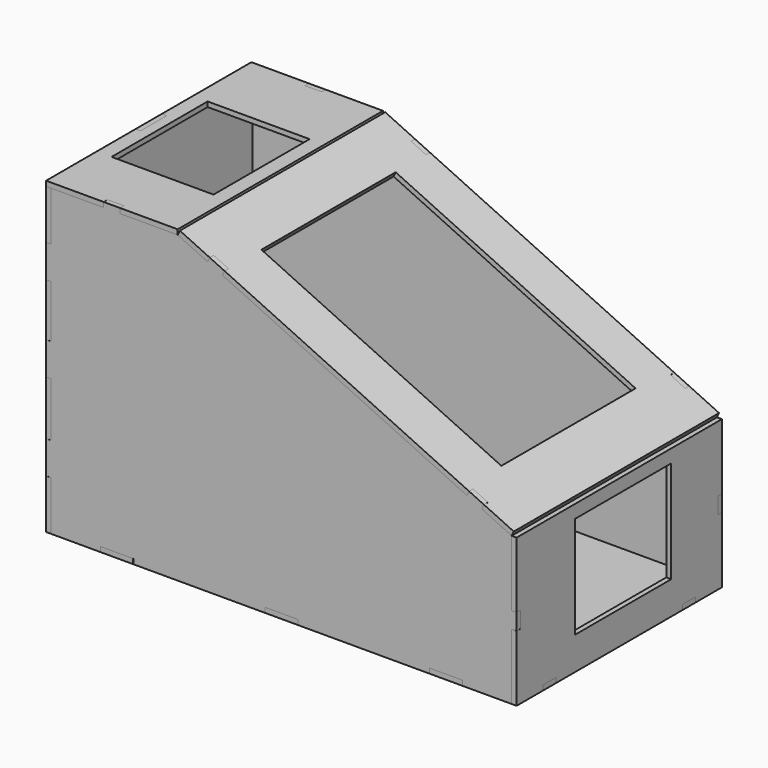
from build123d import *

# Parameters (mm, degrees)
F0_W      = 280
F0_H      = 150
F1_DEPTH  = 3
F2_W      = 73
F2_H      = 62
F2_W_2    = 17
F2_H_2    = 3
F2_W_3    = 96
F3_DEPTH  = 3
F4_W      = 27
F4_H      = 3
F4_W_2    = 66
F4_W_3    = 17
F5_DEPTH  = 3
F6_W      = 3
F6_H      = 68
F6_W_2    = 62
F6_H_2    = 73
F7_DEPTH  = 3
F8_W      = 280
F8_H      = 3
F9_DEPTH  = 3
F10_W     = 280
F10_H     = 3
F11_DEPTH = 3
F12_W     = 20
F12_H     = 3
F12_W_2   = 164.0647657623
F12_W_3   = 161
F12_H_2   = 102
F13_DEPTH = 3
F14_W     = 3
F14_H     = 19.9761795811
F15_DEPTH = 3
F16_W     = 3
F16_H     = 19.9768692255
F16_H_2   = 19.9654474854
F16_H_3   = 19.9758000672
F17_DEPTH = 3
F18_W     = 19.950363785
F18_H     = 3
F18_W_2   = 19.9684463441
F19_DEPTH = 3
F20_W     = 3
F20_H     = 19.9769586325
F20_H_2   = 19.9680477381
F20_H_3   = 19.977606833
F21_DEPTH = 3
F23_W     = 9.9835321307
F23_H     = 3
F24_DEPTH = 3
F25_W     = 9.978748858
F25_H     = 3
F26_DEPTH = 3
F27_W     = 20
F27_H     = 3
F28_DEPTH = 3
F29_W     = 20
F29_H     = 3
F30_DEPTH = 3
F31_W     = 19.9709534645
F31_H     = 3
F31_W_2   = 19.9618935585
F31_W_3   = 19.9760207906
F32_DEPTH = 3
F33_W     = 9.9784359336
F33_H     = 3
F33_W_2   = 9.994674474
F34_DEPTH = 3
F35_W     = 3
F35_H     = 9.9887661636
F36_DEPTH = 3
F37_W     = 3
F37_H     = 9.9958628416
F38_DEPTH = 3
F39_W     = 19.973538816
F39_H     = 3
F39_W_2   = 19.9738545343
F39_W_3   = 19.9763923883
F40_DEPTH = 3
F41_W     = 9.9856257439
F41_H     = 3
F41_W_2   = 9.9614001811
F42_DEPTH = 3
F43_W     = 9.9793635309
F43_H     = 3
F43_W_2   = 9.9839419127
F44_DEPTH = 3


with BuildPart() as f1:
    # F0 (on Top) → F1 (new body)
    with BuildSketch(Plane.XY):
        with Locations((0.3347266465, 5.760698552)):
            Rectangle(F0_W, F0_H)
    extrude(amount=F1_DEPTH)

    # F18 (on face) → F19 (join)
    with BuildSketch(Plane(origin=(-139.6652733535, 0, 0), x_dir=(0, -1, 0), z_dir=(-1, 0, 0))):
        with Locations((-53.7553559989, 1.5)):
            Rectangle(F18_W, F18_H)
        with Locations((32.2464499623, 1.5)):
            Rectangle(F18_W_2, F18_H)
    extrude(amount=F19_DEPTH)

    # F31 (on face) → F32 (join)
    with BuildSketch(Plane.XZ.offset(69.239301448)):
        with Locations((-99.6759831905, 1.5)):
            Rectangle(F31_W, F31_H)
        with Locations((100.318454206, 1.5)):
            Rectangle(F31_W_2, F31_H)
        with Locations((0.3386368044, 1.5)):
            Rectangle(F31_W_3, F31_H)
    extrude(amount=F32_DEPTH)

    # F33 (on face) → F34 (join)
    with BuildSketch(Plane.YZ.offset(140.3347266465)):
        with Locations((-47.2331680357, 1.5)):
            Rectangle(F33_W, F33_H)
        with Locations((58.7589647621, 1.5)):
            Rectangle(F33_W_2, F33_H)
    extrude(amount=F34_DEPTH)

    # F39 (on face) → F40 (join)
    with BuildSketch(Plane(origin=(0, 80.760698552, 0), x_dir=(-1, 0, 0), z_dir=(0, 1, 0))):
        with Locations((99.6645279229, 1.5)):
            Rectangle(F39_W, F39_H)
        with Locations((-0.3459225409, 1.5)):
            Rectangle(F39_W_2, F39_H)
        with Locations((-100.3399789333, 1.5)):
            Rectangle(F39_W_3, F39_H)
    extrude(amount=F40_DEPTH)


with BuildPart() as f3:
    # F2 (on face) → F3 (new body)
    with BuildSketch(Plane.YZ.offset(140.3347266465)):
        Polygon((-72.239301448, 40), (-72.239301448, 0), (-69.239301448, 0), (-69.239301448, 3), (-52.239301448, 3), (-42.239301448, 3), (53.760698552, 3), (63.760698552, 3), (80.760698552, 3), (80.760698552, 0), (83.760698552, 0), (83.760698552, 40), (80.760698552, 40), (80.760698552, 50), (83.760698552, 50), (83.760698552, 90), (-72.239301448, 90), (-72.239301448, 50), (-69.239301448, 50), (-69.239301448, 40), align=None)
        with Locations((8.760698552, 51)):
            Rectangle(F2_W, F2_H, mode=Mode.SUBTRACT)
        with Locations((-60.739301448, 1.5)):
            Rectangle(F2_W_2, F2_H_2)
        with Locations((5.760698552, 1.5)):
            Rectangle(F2_W_3, F2_H_2)
        with Locations((72.260698552, 1.5)):
            Rectangle(F2_W_2, F2_H_2)
    extrude(amount=F3_DEPTH)


with BuildPart() as f5:
    # F4 (on face) → F5 (new body)
    with BuildSketch(Plane(origin=(-139.6652733535, 0, 0), x_dir=(0, -1, 0), z_dir=(-1, 0, 0))):
        Polygon((-83.760698552, 30), (-83.760698552, 0), (-80.760698552, 0), (-80.760698552, 3), (-63.760698552, 3), (-43.760698552, 3), (22.239301448, 3), (42.239301448, 3), (69.239301448, 3), (69.239301448, 0), (72.239301448, 0), (72.239301448, 30), (69.239301448, 30), (69.239301448, 50), (72.239301448, 50), (72.239301448, 83), (69.239301448, 83), (69.239301448, 103), (72.239301448, 103), (72.239301448, 135), (69.239301448, 135), (69.239301448, 155), (72.239301448, 155), (72.239301448, 185), (4.239301448, 185), (-15.760698552, 185), (-83.760698552, 185), (-83.760698552, 155), (-80.760698552, 155), (-80.760698552, 135), (-83.760698552, 135), (-83.760698552, 103), (-80.760698552, 103), (-80.760698552, 83), (-83.760698552, 83), (-83.760698552, 50), (-80.760698552, 50), (-80.760698552, 30), align=None)
        with Locations((55.739301448, 1.5)):
            Rectangle(F4_W, F4_H)
        with Locations((-10.760698552, 1.5)):
            Rectangle(F4_W_2, F4_H)
        with Locations((-72.260698552, 1.5)):
            Rectangle(F4_W_3, F4_H)
    extrude(amount=F5_DEPTH)

    # F14 (on face) → F15 (join)
    with BuildSketch(Plane.XY.offset(185)):
        with Locations((-141.1652733535, 5.7652241085)):
            Rectangle(F14_W, F14_H)
    extrude(amount=F15_DEPTH)


with BuildPart() as f7:
    # F6 (on face) → F7 (new body)
    with BuildSketch(Plane.XY.offset(185)):
        with Locations((-141.1652733535, -38.239301448)):
            Rectangle(F6_W, F6_H)
        with Locations((-141.1652733535, 49.760698552)):
            Rectangle(F6_W, F6_H)
        Polygon((-139.6652733535, -4.239301448), (-139.6652733535, -72.239301448), (-107.6652733535, -72.239301448), (-107.6652733535, -69.239301448), (-97.6652733535, -69.239301448), (-97.6652733535, -72.239301448), (-62.6652733535, -72.239301448), (-62.6652733535, 83.760698552), (-97.6652733535, 83.760698552), (-97.6652733535, 80.760698552), (-107.6652733535, 80.760698552), (-107.6652733535, 83.760698552), (-139.6652733535, 83.760698552), (-139.6652733535, 15.760698552), align=None)
        with Locations((-102.6652733535, 2.760698552)):
            Rectangle(F6_W_2, F6_H_2, mode=Mode.SUBTRACT)
    extrude(amount=F7_DEPTH)


with BuildPart() as f9:
    # F8 (on face) → F9 (new body)
    with BuildSketch(Plane.XZ.offset(69.239301448)):
        Polygon((-139.6652733535, 185), (-139.6652733535, 3), (140.3347266465, 3), (140.3347266465, 90), (-62.6652733535, 185), align=None)
        with Locations((0.3347266465, 1.5)):
            Rectangle(F8_W, F8_H)
    extrude(amount=F9_DEPTH)

    # F16 (on face) → F17 (join)
    with BuildSketch(Plane(origin=(-139.6652733535, 0, 0), x_dir=(0, -1, 0), z_dir=(-1, 0, 0))):
        with Locations((70.739301448, 144.9948176742)):
            Rectangle(F16_W, F16_H)
        with Locations((70.739301448, 92.9838009179)):
            Rectangle(F16_W, F16_H_2)
        with Locations((70.739301448, 39.9933177978)):
            Rectangle(F16_W, F16_H_3)
    extrude(amount=F17_DEPTH)

    # F25 (on face) → F26 (join)
    with BuildSketch(Plane.XY.offset(185)):
        with Locations((-102.6640348136, -70.739301448)):
            Rectangle(F25_W, F25_H)
    extrude(amount=F26_DEPTH)

    # F29 (on face) → F30 (cut)
    with BuildSketch(Plane(origin=(0, 0, 0), x_dir=(1, 0, 0), z_dir=(0, 0, -1))):
        with Locations((100.3347266465, 70.739301448)):
            Rectangle(F29_W, F29_H)
        with Locations((0.3347266465, 70.739301448)):
            Rectangle(F29_W, F29_H)
        with Locations((-99.6652733535, 70.739301448)):
            Rectangle(F29_W, F29_H)
    extrude(amount=-F30_DEPTH, mode=Mode.SUBTRACT)

    # F35 (on face) → F36 (join)
    with BuildSketch(Plane.YZ.offset(140.3347266465)):
        with Locations((-70.739301448, 45.0031179935)):
            Rectangle(F35_W, F35_H)
    extrude(amount=F36_DEPTH)

    # F41 (on face) → F42 (join)
    with BuildSketch(Plane(origin=(59.7637239317, 0, 127.7056416646), x_dir=(0.9057266724, 0, -0.4238622358), z_dir=(0.4238622358, 0, 0.9057266724))):
        with Locations((-110.1135164499, -70.739301448)):
            Rectangle(F41_W, F41_H)
        with Locations((63.9471765608, -70.739301448)):
            Rectangle(F41_W_2, F41_H)
    extrude(amount=F42_DEPTH)


with BuildPart() as f11:
    # F10 (on face) → F11 (new body)
    with BuildSketch(Plane(origin=(0, 80.760698552, 0), x_dir=(-1, 0, 0), z_dir=(0, 1, 0))):
        Polygon((-140.3347266465, 90), (-140.3347266465, 3), (139.6652733535, 3), (139.6652733535, 185), (62.6652733535, 185), align=None)
        with Locations((-0.3347266465, 1.5)):
            Rectangle(F10_W, F10_H)
    extrude(amount=F11_DEPTH)

    # F20 (on face) → F21 (join)
    with BuildSketch(Plane(origin=(-139.6652733535, 0, 0), x_dir=(0, -1, 0), z_dir=(-1, 0, 0))):
        with Locations((-82.260698552, 145.0085863471)):
            Rectangle(F20_W, F20_H)
        with Locations((-82.260698552, 92.994004488)):
            Rectangle(F20_W, F20_H_2)
        with Locations((-82.260698552, 40.001526475)):
            Rectangle(F20_W, F20_H_3)
    extrude(amount=F21_DEPTH)

    # F22: union 

    # F23 (on face) → F24 (join)
    with BuildSketch(Plane.XY.offset(185)):
        with Locations((-102.6701591909, 82.260698552)):
            Rectangle(F23_W, F23_H)
    extrude(amount=F24_DEPTH)

    # F27 (on face) → F28 (cut)
    with BuildSketch(Plane(origin=(0, 0, 0), x_dir=(1, 0, 0), z_dir=(0, 0, -1))):
        with Locations((-99.6652733535, -82.260698552)):
            Rectangle(F27_W, F27_H)
        with Locations((0.3347266465, -82.260698552)):
            Rectangle(F27_W, F27_H)
        with Locations((100.3347266465, -82.260698552)):
            Rectangle(F27_W, F27_H)
    extrude(amount=-F28_DEPTH, mode=Mode.SUBTRACT)

    # F37 (on face) → F38 (join)
    with BuildSketch(Plane.YZ.offset(140.3347266465)):
        with Locations((82.260698552, 45.0009405613)):
            Rectangle(F37_W, F37_H)
    extrude(amount=F38_DEPTH)

    # F43 (on face) → F44 (join)
    with BuildSketch(Plane(origin=(59.7637239317, 0, 127.7056416646), x_dir=(0.9057266724, 0, -0.4238622358), z_dir=(0.4238622358, 0, 0.9057266724))):
        with Locations((63.9634002, 82.260698552)):
            Rectangle(F43_W, F43_H)
        with Locations((-110.1040318608, 82.260698552)):
            Rectangle(F43_W_2, F43_H)
    extrude(amount=F44_DEPTH)


with BuildPart() as f13:
    # F12 (on face) → F13 (new body)
    with BuildSketch(Plane(origin=(59.7637239317, 0, 127.7056416646), x_dir=(0.9057266724, 0, -0.4238622358), z_dir=(0.4238622358, 0, 0.9057266724))):
        with Locations((78.9573037575, -70.739301448)):
            Rectangle(F12_W, F12_H)
        with Locations((-23.0750791236, -70.739301448)):
            Rectangle(F12_W_2, F12_H)
        with Locations((-125.1074620047, -70.739301448)):
            Rectangle(F12_W, F12_H)
        Polygon((68.9573037575, -69.239301448), (88.9573037575, -69.239301448), (88.9573037575, 83.760698552), (68.9573037575, 83.760698552), (68.9573037575, 80.760698552), (58.9573037575, 80.760698552), (58.9573037575, 83.760698552), (-105.1074620047, 83.760698552), (-105.1074620047, 80.760698552), (-115.1074620047, 80.760698552), (-115.1074620047, 83.760698552), (-135.1074620047, 83.760698552), (-135.1074620047, -69.239301448), (-115.1074620047, -69.239301448), (-105.1074620047, -69.239301448), (58.9573037575, -69.239301448), align=None)
        with Locations((-24.6074620047, 6.760698552)):
            Rectangle(F12_W_3, F12_H_2, mode=Mode.SUBTRACT)
    extrude(amount=F13_DEPTH)


solid = Compound([f1.part, f3.part, f5.part, f7.part, f9.part, f11.part, f13.part])
